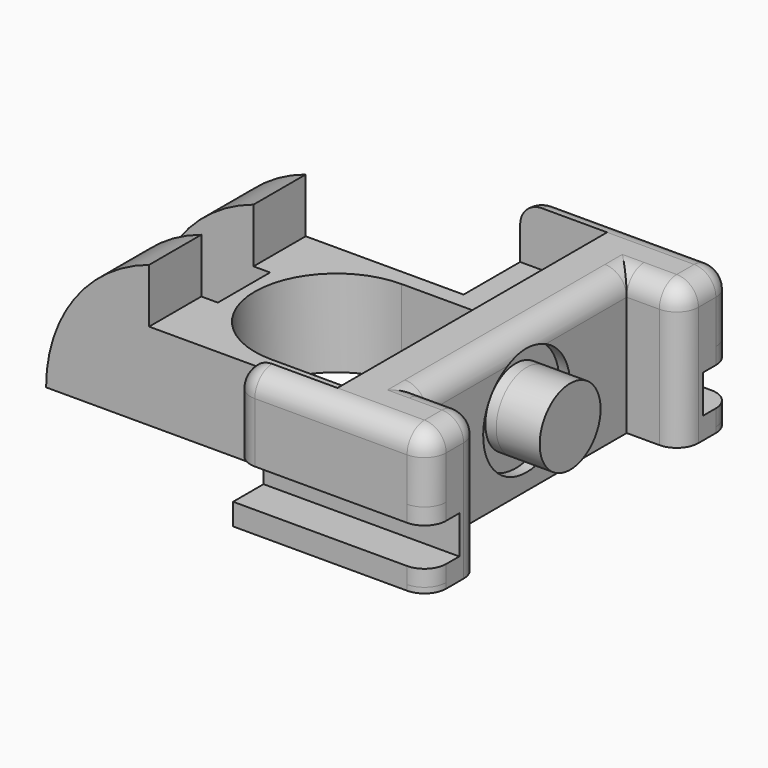
from build123d import *
from build123d import SkipClean  # not in build123d's __all__

# Parameters (mm, degrees)
F0_W          = 10
F0_H          = 6
F1_DEPTH      = 13
F3_DEPTH      = 25
F4_W          = 22.5231910496
F4_H          = 31
F5_DEPTH      = 5
F7_DEPTH      = 8
F8_R          = 5
F8_R_2        = 3.5
F9_DEPTH      = 1
F10_DEPTH     = 4
F11_W         = 3.5
F11_H         = 3.5
F12_DEPTH     = 42.001
F13_W         = 3.5
F13_H         = 3.5
F14_DEPTH     = 42.001
F15_T1_DEPTH  = 14
F15_T3_DEPTH  = 2
F15_T5_DEPTH  = 3
F15_T7_DEPTH  = 23
F15_T9_DEPTH  = 2
F15_T11_DEPTH = 10.5
F15_T13_DEPTH = 12
F15_T15_DEPTH = 16
F15_T17_DEPTH = 5.5
F15_S21_W     = 2.04
F15_S21_H     = 2.04
F15_T22_DEPTH = 2.04
F15_S27_W     = 2.04
F15_S27_H     = 2.04
F15_T28_DEPTH = 2.04
F15_S33_W     = 2.04
F15_S33_H     = 2.04
F15_T34_DEPTH = 2.04
F15_S39_W     = 2.04
F15_S39_H     = 2.04
F15_T40_DEPTH = 2.04
F15_S45_W     = 2.04
F15_S45_H     = 2.04
F15_T46_DEPTH = 2.04
F15_S51_W     = 2.04
F15_S51_H     = 2.04
F15_T52_DEPTH = 2.04
F15_T59_DEPTH = 28
F15_T63_DEPTH = 8
F15_T70_DEPTH = 8
F15_T74_DEPTH = 28


# Not quite as in the source:
# - a fillet or chamfer that OpenCascade refuses, or shapes differently, is made with other operations: its cross-section is extruded or revolved along the edge and cut away or added


with BuildPart() as f1:
    # F0 (on Top) → F1 (new body)
    with BuildSketch(Plane.XY):
        with Locations((-34.8019978553, 9)):
            Rectangle(F0_W, F0_H)
        with Locations((-34.8019978553, -3)):
            Rectangle(F0_W, F0_H)
        Polygon((2.1980021447, 20.5), (-15.8019978553, 20.5), (-15.8019978553, 12), (-29.8019978553, 12), (-29.8019978553, 6), (-28.8019978553, 6), (-28.8019978553, 0), (-29.8019978553, 0), (-29.8019978553, -6), (-15.8019978553, -6), (-15.8019978553, -14.5), (2.1980021447, -14.5), (2.1980021447, -8.5), (-2.8019978553, -8.5), (-2.8019978553, 14.5), (2.1980021447, 14.5), align=None)
    extrude(amount=F1_DEPTH)

    # F2 (on face) → F3 (cut)
    with BuildSketch(Plane.XZ.offset(6)):
        with BuildLine():
            Line((-39.8019978553, 13), (-39.8019978553, 0))
            ThreePointArc((-39.8019978553, 0), (-37.1813109556, 8.0437849903), (-30.3251889049, 13))
            Line((-30.3251889049, 13), (-39.8019978553, 13))
        make_face()
    extrude(amount=-F3_DEPTH, mode=Mode.SUBTRACT)

    # F4 (on face) → F5 (cut)
    with BuildSketch(Plane.XY.offset(13)):
        with Locations((-19.0635933801, 3)):
            Rectangle(F4_W, F4_H)
    extrude(amount=-F5_DEPTH, mode=Mode.SUBTRACT)

    # F6 (on face) → F7 (cut, through all)
    with BuildSketch(Plane(origin=(0, 0, 0), x_dir=(1, 0, 0), z_dir=(0, 0, -1))):
        with BuildLine():
            Line((-11.8019978553, 4.5), (-20.3019978553, 4.5))
            ThreePointArc((-20.3019978553, 4.5), (-27.8019978553, -3), (-20.3019978553, -10.5))
            Line((-20.3019978553, -10.5), (-11.8019978553, -10.5))
            ThreePointArc((-11.8019978553, -10.5), (-4.3019978553, -3), (-11.8019978553, 4.5))
        make_face()
    extrude(amount=-F7_DEPTH, mode=Mode.SUBTRACT)

    # F8 (on face) → F9 (cut)
    with BuildSketch(Plane.YZ.offset(-2.8019978553)):
        with Locations((3, 6.5)):
            Circle(F8_R)
        with Locations((3, 6.5)):
            Circle(F8_R_2, mode=Mode.SUBTRACT)
    extrude(amount=-F9_DEPTH, mode=Mode.SUBTRACT)

    # F10 (add): a face of the model
    f10_faces = [f1.faces().sort_by_distance(p)[0] for p in [
        (-2.8019978553, 3, 6.5),
    ]]
    extrude(f10_faces, amount=F10_DEPTH)

    # F11 (on face) → F12 (cut, through all)
    with BuildSketch(Plane.YZ.offset(2.1980021447)):
        with Locations((-12.75, 3.75)):
            Rectangle(F11_W, F11_H)
    extrude(amount=-F12_DEPTH, mode=Mode.SUBTRACT)

    # F13 (on face) → F14 (cut, through all)
    with BuildSketch(Plane.YZ.offset(2.1980021447)):
        with Locations((18.75, 3.75)):
            Rectangle(F13_W, F13_H)
    extrude(amount=-F14_DEPTH, mode=Mode.SUBTRACT)

    # F15: fillet of radius 2 on 18 edges, made by hand

    # F15_s2 → F15_t1 (cut)
    with BuildSketch(Plane.YZ.offset(-13.8019978553)):
        with BuildLine():
            ThreePointArc((-12.5, 13), (-13.9142135624, 12.4142135624), (-14.5, 11))
            Line((-14.5, 11), (-14.5, 13))
            Line((-14.5, 13), (-12.5, 13))
        make_face()
        with BuildLine():
            ThreePointArc((18.5, 13), (19.9142135624, 12.4142135624), (20.5, 11))
            Line((20.5, 11), (20.5, 13))
            Line((20.5, 13), (18.5, 13))
        make_face()
    extrude(amount=F15_T1_DEPTH, mode=Mode.SUBTRACT)

    # F15_s4 → F15_t3 (cut)
    with BuildSketch(Plane.XZ.offset(10.5)):
        with BuildLine():
            ThreePointArc((2.1980021447, 11), (1.6122157071, 12.4142135624), (0.1980021447, 13))
            Line((0.1980021447, 13), (2.1980021447, 13))
            Line((2.1980021447, 13), (2.1980021447, 11))
        make_face()
    extrude(amount=F15_T3_DEPTH, mode=Mode.SUBTRACT)

    # F15_s6 → F15_t5 (cut)
    with BuildSketch(Plane.YZ.offset(-2.8019978553)):
        with BuildLine():
            ThreePointArc((-8.5, 11), (-9.0857864376, 12.4142135624), (-10.5, 13))
            Line((-10.5, 13), (-8.5, 13))
            Line((-8.5, 13), (-8.5, 11))
        make_face()
        with BuildLine():
            ThreePointArc((14.5, 11), (15.0857864376, 12.4142135624), (16.5, 13))
            Line((16.5, 13), (14.5, 13))
            Line((14.5, 13), (14.5, 11))
        make_face()
    extrude(amount=F15_T5_DEPTH, mode=Mode.SUBTRACT)

    # F15_s8 → F15_t7 (cut)
    with BuildSketch(Plane.XZ.offset(-14.5)):
        with BuildLine():
            ThreePointArc((-2.8019978553, 11), (-3.3877842929, 12.4142135624), (-4.8019978553, 13))
            Line((-4.8019978553, 13), (-2.8019978553, 13))
            Line((-2.8019978553, 13), (-2.8019978553, 11))
        make_face()
    extrude(amount=F15_T7_DEPTH, mode=Mode.SUBTRACT)

    # F15_s10 → F15_t9 (cut)
    with BuildSketch(Plane.XZ.offset(-18.5)):
        with BuildLine():
            ThreePointArc((2.1980021447, 11), (1.6122157071, 12.4142135624), (0.1980021447, 13))
            Line((0.1980021447, 13), (2.1980021447, 13))
            Line((2.1980021447, 13), (2.1980021447, 11))
        make_face()
    extrude(amount=F15_T9_DEPTH, mode=Mode.SUBTRACT)

    # F15_s12 → F15_t11 (cut)
    with BuildSketch(Plane.XY.offset(0.5)):
        with BuildLine():
            ThreePointArc((2.1980021447, 18.5), (1.6122157071, 19.9142135624), (0.1980021447, 20.5))
            Line((0.1980021447, 20.5), (2.1980021447, 20.5))
            Line((2.1980021447, 20.5), (2.1980021447, 18.5))
        make_face()
        with BuildLine():
            ThreePointArc((-15.8019978553, 18.5), (-15.2162114177, 19.9142135624), (-13.8019978553, 20.5))
            Line((-13.8019978553, 20.5), (-15.8019978553, 20.5))
            Line((-15.8019978553, 20.5), (-15.8019978553, 18.5))
        make_face()
        with BuildLine():
            ThreePointArc((2.1980021447, -12.5), (1.6122157071, -13.9142135624), (0.1980021447, -14.5))
            Line((0.1980021447, -14.5), (2.1980021447, -14.5))
            Line((2.1980021447, -14.5), (2.1980021447, -12.5))
        make_face()
    extrude(amount=F15_T11_DEPTH, mode=Mode.SUBTRACT)

    # F15_s14 → F15_t13 (cut)
    with BuildSketch(Plane.XY.offset(-5)):
        with BuildLine():
            ThreePointArc((-15.8019978553, 18.5), (-15.2162114177, 19.9142135624), (-13.8019978553, 20.5))
            Line((-13.8019978553, 20.5), (-15.8019978553, 20.5))
            Line((-15.8019978553, 20.5), (-15.8019978553, 18.5))
        make_face()
        with BuildLine():
            ThreePointArc((0.1980021447, -14.5), (1.6122157071, -13.9142135624), (2.1980021447, -12.5))
            Line((2.1980021447, -12.5), (2.1980021447, -14.5))
            Line((2.1980021447, -14.5), (0.1980021447, -14.5))
        make_face()
        with BuildLine():
            ThreePointArc((0.1980021447, 20.5), (1.6122157071, 19.9142135624), (2.1980021447, 18.5))
            Line((2.1980021447, 18.5), (2.1980021447, 20.5))
            Line((2.1980021447, 20.5), (0.1980021447, 20.5))
        make_face()
    with SkipClean():  # cleaning this boolean's faces spoils the solid; the shape is the same uncleaned
        extrude(amount=F15_T13_DEPTH, mode=Mode.SUBTRACT)

    # F15_s16 → F15_t15 (cut)
    with BuildSketch(Plane.XY.offset(-5)):
        with BuildLine():
            ThreePointArc((0.1980021447, -8.5), (1.6122157071, -9.0857864376), (2.1980021447, -10.5))
            Line((2.1980021447, -10.5), (2.1980021447, -8.5))
            Line((2.1980021447, -8.5), (0.1980021447, -8.5))
        make_face()
        with BuildLine():
            ThreePointArc((2.1980021447, 16.5), (1.6122157071, 15.0857864376), (0.1980021447, 14.5))
            Line((0.1980021447, 14.5), (2.1980021447, 14.5))
            Line((2.1980021447, 14.5), (2.1980021447, 16.5))
        make_face()
    extrude(amount=F15_T15_DEPTH, mode=Mode.SUBTRACT)

    # F15_s18 → F15_t17 (cut)
    with BuildSketch(Plane.XY.offset(5.5)):
        with BuildLine():
            ThreePointArc((-15.8019978553, -12.5), (-15.2162114177, -13.9142135624), (-13.8019978553, -14.5))
            Line((-13.8019978553, -14.5), (-15.8019978553, -14.5))
            Line((-15.8019978553, -14.5), (-15.8019978553, -12.5))
        make_face()
    extrude(amount=F15_T17_DEPTH, mode=Mode.SUBTRACT)


with BuildPart() as f15_tool20:
    # F15_s21 → F15_t22 (new body)
    with BuildSketch(Plane.XY.offset(11)):
        with Locations((-14.8219978553, -13.52)):
            Rectangle(F15_S21_W, F15_S21_H)
    extrude(amount=F15_T22_DEPTH)

    # F15_s23 → F15_t24 (revolve, cut)
    with BuildSketch(Plane(origin=(-13.8019978553, -12.5, 11), x_dir=(0.7071067812, 0.7071067812, 0), z_dir=(0.7071067812, -0.7071067812, 0))):
        with BuildLine():
            ThreePointArc((0, -2), (2, 0), (0, 2))
            Line((0, 2), (0, -2))
        make_face()
    revolve(axis=Axis((-13.8019978553, -12.5, 11), (0, 0, 1)), mode=Mode.SUBTRACT)


with BuildPart() as f1_1:
    add(f1.part, clean=False)

    # F15_t19: cut F15_tool20
    add(f15_tool20.part, mode=Mode.SUBTRACT)


with BuildPart() as f15_tool26:
    # F15_s27 → F15_t28 (new body)
    with BuildSketch(Plane.XY.offset(11)):
        with Locations((1.2180021447, -13.52)):
            Rectangle(F15_S27_W, F15_S27_H)
    extrude(amount=F15_T28_DEPTH)

    # F15_s29 → F15_t30 (revolve, cut)
    with BuildSketch(Plane(origin=(0.1980021447, -12.5, 11), x_dir=(-0.7071067812, 0.7071067812, 0), z_dir=(0.7071067812, 0.7071067812, 0))):
        with BuildLine():
            ThreePointArc((0, -2), (2, 0), (0, 2))
            Line((0, 2), (0, -2))
        make_face()
    revolve(axis=Axis((0.1980021447, -12.5, 11), (0, 0, 1)), mode=Mode.SUBTRACT)


with BuildPart() as f1_2:
    add(f1_1.part, clean=False)

    # F15_t25: cut F15_tool26
    add(f15_tool26.part, mode=Mode.SUBTRACT)


with BuildPart() as f15_tool32:
    # F15_s33 → F15_t34 (new body)
    with BuildSketch(Plane.YZ.offset(0.1980021447)):
        with Locations((-9.48, 12.02)):
            Rectangle(F15_S33_W, F15_S33_H)
    extrude(amount=F15_T34_DEPTH)

    # F15_s35 → F15_t36 (revolve, cut)
    with BuildSketch(Plane(origin=(0.1980021447, -10.5, 11), x_dir=(0, -0.7071067812, -0.7071067812), z_dir=(0, -0.7071067812, 0.7071067812))):
        with BuildLine():
            ThreePointArc((0, -2), (2, 0), (0, 2))
            Line((0, 2), (0, -2))
        make_face()
    revolve(axis=Axis((0.1980021447, -10.5, 11), (1, 0, 0)), mode=Mode.SUBTRACT)


with BuildPart() as f1_3:
    add(f1_2.part, clean=False)

    # F15_t31: cut F15_tool32
    add(f15_tool32.part, mode=Mode.SUBTRACT)


with BuildPart() as f15_tool38:
    # F15_s39 → F15_t40 (new body)
    with BuildSketch(Plane.XY.offset(11)):
        with Locations((1.2180021447, 15.48)):
            Rectangle(F15_S39_W, F15_S39_H)
    extrude(amount=F15_T40_DEPTH)

    # F15_s41 → F15_t42 (revolve, cut)
    with BuildSketch(Plane(origin=(0.1980021447, 16.5, 11), x_dir=(-0.7071067812, 0.7071067812, 0), z_dir=(0.7071067812, 0.7071067812, 0))):
        with BuildLine():
            ThreePointArc((0, -2), (2, 0), (0, 2))
            Line((0, 2), (0, -2))
        make_face()
    revolve(axis=Axis((0.1980021447, 16.5, 11), (0, 0, 1)), mode=Mode.SUBTRACT)


with BuildPart() as f1_4:
    add(f1_3.part, clean=False)

    # F15_t37: cut F15_tool38
    add(f15_tool38.part, mode=Mode.SUBTRACT)


with BuildPart() as f15_tool44:
    # F15_s45 → F15_t46 (new body)
    with BuildSketch(Plane.XY.offset(11)):
        with Locations((1.2180021447, 19.52)):
            Rectangle(F15_S45_W, F15_S45_H)
    extrude(amount=F15_T46_DEPTH)

    # F15_s47 → F15_t48 (revolve, cut)
    with BuildSketch(Plane(origin=(0.1980021447, 18.5, 11), x_dir=(-0.7071067812, -0.7071067812, 0), z_dir=(-0.7071067812, 0.7071067812, 0))):
        with BuildLine():
            ThreePointArc((0, -2), (2, 0), (0, 2))
            Line((0, 2), (0, -2))
        make_face()
    revolve(axis=Axis((0.1980021447, 18.5, 11), (0, 0, 1)), mode=Mode.SUBTRACT)


with BuildPart() as f1_5:
    add(f1_4.part, clean=False)

    # F15_t43: cut F15_tool44
    add(f15_tool44.part, mode=Mode.SUBTRACT)


with BuildPart() as f15_tool50:
    # F15_s51 → F15_t52 (new body)
    with BuildSketch(Plane.XY.offset(11)):
        with Locations((-14.8219978553, 19.52)):
            Rectangle(F15_S51_W, F15_S51_H)
    extrude(amount=F15_T52_DEPTH)

    # F15_s53 → F15_t54 (revolve, cut)
    with BuildSketch(Plane(origin=(-13.8019978553, 18.5, 11), x_dir=(0.7071067812, -0.7071067812, 0), z_dir=(-0.7071067812, -0.7071067812, 0))):
        with BuildLine():
            ThreePointArc((0, -2), (2, 0), (0, 2))
            Line((0, 2), (0, -2))
        make_face()
    revolve(axis=Axis((-13.8019978553, 18.5, 11), (0, 0, 1)), mode=Mode.SUBTRACT)


with BuildPart() as f1_6:
    add(f1_5.part, clean=False)

    # F15_t49: cut F15_tool50
    add(f15_tool50.part, mode=Mode.SUBTRACT)


with BuildPart() as f15_tool57:
    # F15_s58 → F15_t59 (new body)
    with BuildSketch(Plane.XZ.offset(13.5)):
        with BuildLine():
            ThreePointArc((-2.8019978553, 11), (-3.3877842929, 12.4142135624), (-4.8019978553, 13))
            Line((-4.8019978553, 13), (-2.8019978553, 13))
            Line((-2.8019978553, 13), (-2.8019978553, 11))
        make_face()
    extrude(amount=-F15_T59_DEPTH)

    split(bisect_by=Plane.XZ.offset(8.5), keep=Keep.TOP)


with BuildPart() as f15_tool61:
    # F15_s62 → F15_t63 (new body)
    with BuildSketch(Plane.YZ.offset(0.1980021447)):
        with BuildLine():
            ThreePointArc((-8.5, 11), (-9.0857864376, 12.4142135624), (-10.5, 13))
            Line((-10.5, 13), (-8.5, 13))
            Line((-8.5, 13), (-8.5, 11))
        make_face()
    extrude(amount=-F15_T63_DEPTH)

    split(bisect_by=Plane.YZ.offset(-2.8019978553), keep=Keep.BOTTOM)


with BuildPart() as f15_tool57_1:
    add(f15_tool57.part, clean=False)

    # F15_t65: intersect F15_tool61
    add(f15_tool61.part, mode=Mode.INTERSECT)


with BuildPart() as f1_7:
    add(f1_6.part, clean=False)

    # F15_t55: cut F15_tool57
    add(f15_tool57_1.part, mode=Mode.SUBTRACT)


with BuildPart() as f15_tool68:
    # F15_s69 → F15_t70 (new body)
    with BuildSketch(Plane.YZ.offset(-7.8019978553)):
        with BuildLine():
            ThreePointArc((14.5, 11), (15.0857864376, 12.4142135624), (16.5, 13))
            Line((16.5, 13), (14.5, 13))
            Line((14.5, 13), (14.5, 11))
        make_face()
    extrude(amount=F15_T70_DEPTH)

    split(bisect_by=Plane.YZ.offset(-2.8019978553), keep=Keep.BOTTOM)


with BuildPart() as f15_tool72:
    # F15_s73 → F15_t74 (new body)
    with BuildSketch(Plane.XZ.offset(8.5)):
        with BuildLine():
            ThreePointArc((-2.8019978553, 11), (-3.3877842929, 12.4142135624), (-4.8019978553, 13))
            Line((-4.8019978553, 13), (-2.8019978553, 13))
            Line((-2.8019978553, 13), (-2.8019978553, 11))
        make_face()
    extrude(amount=-F15_T74_DEPTH)

    split(bisect_by=Plane.XZ.offset(-14.5), keep=Keep.BOTTOM)


with BuildPart() as f15_tool68_1:
    add(f15_tool68.part, clean=False)

    # F15_t76: intersect F15_tool72
    add(f15_tool72.part, mode=Mode.INTERSECT)


with BuildPart() as f1_8:
    add(f1_7.part, clean=False)

    # F15_t66: cut F15_tool68
    add(f15_tool68_1.part, mode=Mode.SUBTRACT)


solid = f1_8.part
